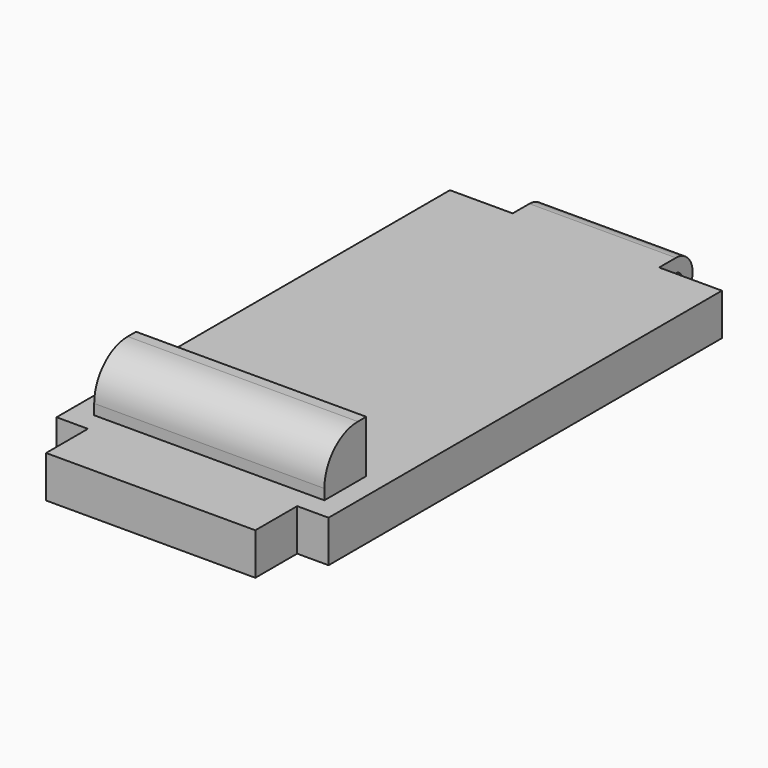
from build123d import *

# Parameters (mm, degrees)
F0_W      = 33.02
F0_H      = 59.69
F1_DEPTH  = 5.08
F2_W      = 17.78
F2_H      = 5.08
F3_DEPTH  = 5.08
F4_R      = 0.889
F5_DEPTH  = 17.78
F6_R      = 2.53999
F7_W      = 27.94
F7_H      = 6.35
F8_DEPTH  = 6.35
F9_R      = 5.08
F10_W     = 25.4
F10_H     = 5.08
F11_DEPTH = 6.35


# Not quite as in the source:
# - a fillet or chamfer is up to 0.001 mm smaller than in the source, because OpenCascade refuses the exact size


with BuildPart() as f1:
    # F0 (on Top) → F1 (new body)
    with BuildSketch(Plane.XY):
        with Locations((16.51, 29.845)):
            Rectangle(F0_W, F0_H)
    extrude(amount=F1_DEPTH)

    # F2 (on face) → F3 (join)
    with BuildSketch(Plane(origin=(0, 59.69, 0), x_dir=(-1, 0, 0), z_dir=(0, 1, 0))):
        with Locations((-16.51, 2.54)):
            Rectangle(F2_W, F2_H)
    extrude(amount=F3_DEPTH)

    # F4 (on face) → F5 (cut)
    with BuildSketch(Plane(origin=(7.62, 0, 0), x_dir=(0, -1, 0), z_dir=(-1, 0, 0))):
        with Locations((-62.23, 2.54)):
            Circle(F4_R)
    extrude(amount=-F5_DEPTH, mode=Mode.SUBTRACT)

    # F6 (radius 2.54 in the source; OpenCascade refuses exactly that, so slightly less here)
    f6_edges = [f1.edges().sort_by_distance(p)[0] for p in [
        (16.51, 64.77, 0),
        (16.51, 64.77, 5.08),
    ]]
    fillet(f6_edges, radius=F6_R)

    # F7 (on face) → F8 (join)
    with BuildSketch(Plane.XY.offset(5.08)):
        with Locations((16.51, 5.715)):
            Rectangle(F7_W, F7_H)
    extrude(amount=F8_DEPTH)

    # F9
    f9_edges = [f1.edges().sort_by_distance(p)[0] for p in [
        (16.51, 2.54, 11.43),
    ]]
    fillet(f9_edges, radius=F9_R)

    # F10 (on face) → F11 (join)
    with BuildSketch(Plane.XZ):
        with Locations((16.51, 2.54)):
            Rectangle(F10_W, F10_H)
    extrude(amount=F11_DEPTH)


solid = f1.part
